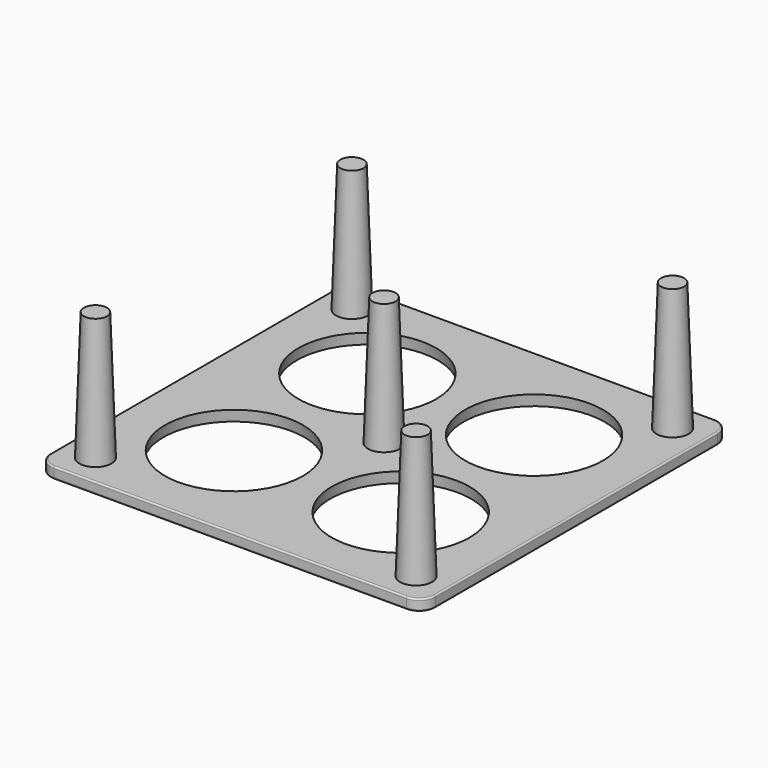
from build123d import *

# Parameters (mm, degrees)
F0_W     = 120
F0_H     = 120
F0_R     = 5
F0_R_2   = 21.5
F1_DEPTH = 3.5
F2_DEPTH = 40
F2_TAPER = 2
F3_R     = 5
F4_SIZE2 = 3.49999
F4_SIZE  = 0.49999
F5_R     = 0.5


# Not quite as in the source:
# - a fillet or chamfer is up to 0.001 mm smaller than in the source, because OpenCascade refuses the exact size


with BuildPart() as f1:
    # F0 (on Top) → F1 (new body)
    with BuildSketch(Plane.XY):
        Rectangle(F0_W, F0_H)
        with Locations((-50, -50)):
            Circle(F0_R, mode=Mode.SUBTRACT)
        with Locations((-26, -26)):
            Circle(F0_R_2, mode=Mode.SUBTRACT)
        with Locations((50, -50)):
            Circle(F0_R, mode=Mode.SUBTRACT)
        with Locations((26, -26)):
            Circle(F0_R_2, mode=Mode.SUBTRACT)
        with Locations((-26, 26)):
            Circle(F0_R_2, mode=Mode.SUBTRACT)
        with Locations((-50, 50)):
            Circle(F0_R, mode=Mode.SUBTRACT)
        Circle(F0_R, mode=Mode.SUBTRACT)
        with Locations((26, 26)):
            Circle(F0_R_2, mode=Mode.SUBTRACT)
        with Locations((50, 50)):
            Circle(F0_R, mode=Mode.SUBTRACT)
        with Locations((-50, 50)):
            Circle(F0_R)
        Circle(F0_R)
        with Locations((50, 50)):
            Circle(F0_R)
        with Locations((-50, -50)):
            Circle(F0_R)
        with Locations((50, -50)):
            Circle(F0_R)
    extrude(amount=-F1_DEPTH)

    # F0 (on Top) → F2 (join)
    with BuildSketch(Plane.XY):
        with Locations((-50, 50)):
            Circle(F0_R)
        Circle(F0_R)
        with Locations((50, 50)):
            Circle(F0_R)
        with Locations((50, -50)):
            Circle(F0_R)
        with Locations((-50, -50)):
            Circle(F0_R)
    extrude(amount=F2_DEPTH, taper=F2_TAPER)

    # F3
    f3_edges = [f1.edges().sort_by_distance(p)[0] for p in [
        (-60, -60, -1.75),
        (-60, 60, -1.75),
        (60, 60, -1.75),
        (60, -60, -1.75),
    ]]
    fillet(f3_edges, radius=F3_R)

    # F4 (size 0.5 and 3.5 in the source; OpenCascade refuses exactly that, so slightly less here)
    f4_edges = [f1.edges().sort_by_distance(p)[0] for p in [
        (4.5, 26, -3.5),
        (-47.5, 26, -3.5),
        (-47.5, -26, -3.5),
        (4.5, -26, -3.5),
    ]]
    f4_side = f1.faces().sort_by_distance((0, 0, -3.5))[0]
    chamfer(f4_edges, length=F4_SIZE, length2=F4_SIZE2, reference=f4_side)

    # F5
    f5_edges = [f1.edges().sort_by_distance(p)[0] for p in [
        (0, -60, -3.5),
        (0, -60, 0),
    ]]
    fillet(f5_edges, radius=F5_R)


solid = f1.part
